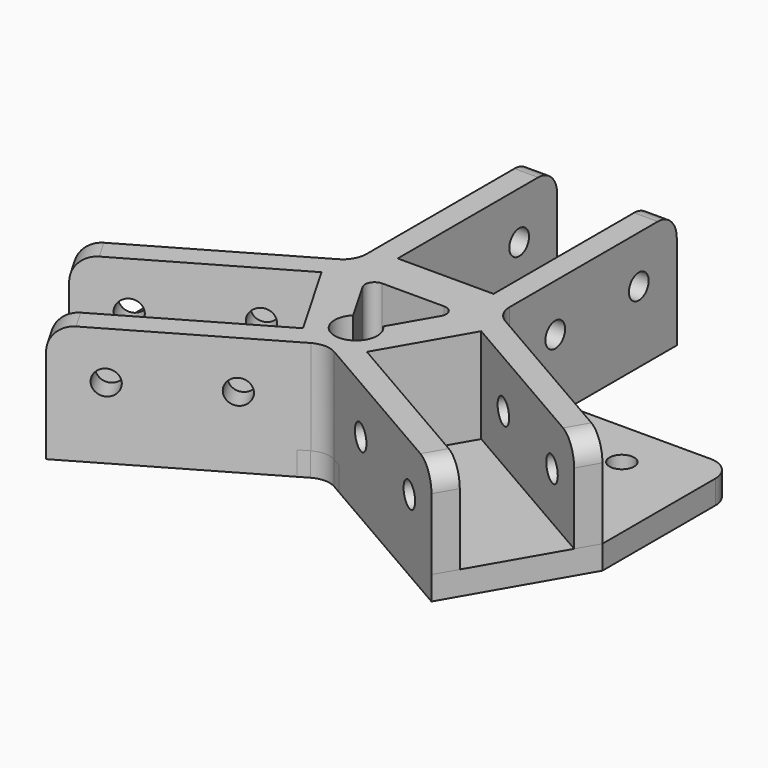
from build123d import *

# Parameters (mm, degrees)
F1_DEPTH    = 20
F2_R        = 2.6
F3_DEPTH    = 50.6016350946
F4_COUNT    = 3
F4_ANGLE    = 240
F6_DEPTH    = 5
F7_T1_DEPTH = 25
F10_DEPTH   = 5
F11_DEPTH   = 25.001
F12_R       = 2
F13_R       = 2.6
F14_DEPTH   = 25.001
F15_R       = 5
F16_R       = 4.5
F17_DEPTH   = 20


# Not quite as in the source:
# - a fillet or chamfer that OpenCascade refuses, or shapes differently, is made with other operations: its cross-section is extruded or revolved along the edge and cut away or added


with BuildPart() as f1:
    # F0 (on Top) → F1 (new body)
    with BuildSketch(Plane.XY):
        Polygon((43.0992290895, -36.5458269543), (6.7261621305, -15.5458269543), (16.8261621305, 1.9478862021), (53.1992290895, -19.0521137979), (55.6992290895, -14.7219867789), (14.8979589003, 8.8346375481), (0, 0), (-0.2020410997, -17.3193296462), (40.5992290895, -40.8759539732), align=None)
    extrude(amount=F1_DEPTH)

    # F2 (on face) → F3 (cut, through all)
    with BuildSketch(Plane(origin=(-7.55, -13.0769835971, 0), x_dir=(0.8660254038, -0.5, 0), z_dir=(-0.5, -0.8660254038, 0))):
        with Locations((45.5979407522, 10)):
            Circle(F2_R)
        with Locations((23.5979407522, 10)):
            Circle(F2_R)
    extrude(amount=-F3_DEPTH, mode=Mode.SUBTRACT)

    # F4: F1 ×3 about axis
    f4_axis = Axis((0, 0, 10), (0, 0, -1))


with BuildPart() as f1_1:
    add(f1.part)
    for i in range(1, F4_COUNT):
        add(f1.part.rotate(f4_axis, i * F4_ANGLE / (F4_COUNT - 1)))

    # F5 (on face) → F6 (join)
    with BuildSketch(Plane(origin=(0, 0, 0), x_dir=(1, 0, 0), z_dir=(0, 0, -1))):
        Polygon((0, 17.4359781295), (-40.5992290895, 40.8759539732), (-55.6992290895, 14.7219867789), (-15.1, -8.7179890648), (-15.1, -55.5979407522), (15.1, -55.5979407522), (15.1, -8.7179890648), (55.6992290895, 14.7219867789), (40.5992290895, 40.8759539732), align=None)
    extrude(amount=F6_DEPTH)

    # F7: fillet of radius 5 on 3 edges, made by hand

    # F7_s2 → F7_t1 (join)
    with BuildSketch(Plane.XY.offset(-5)):
        with BuildLine():
            ThreePointArc((2.5012, -18.8795847426), (0, -18.2093902225), (-2.5012, -18.8795847426))
            Line((-2.5012, -18.8795847426), (-2.75132, -18.4463641946))
            ThreePointArc((-2.75132, -18.4463641946), (-1.50062, -17.7247340932), (-0.25012, -17.0027575815))
            Line((-0.25012, -17.0027575815), (0.25012, -17.0027575815))
            ThreePointArc((0.25012, -17.0027575815), (1.50062, -17.7247340932), (2.75132, -18.4463641946))
            Line((2.75132, -18.4463641946), (2.5012, -18.8795847426))
        make_face()
        with BuildLine():
            ThreePointArc((15.0996, 11.6058951112), (15.7697945201, 9.1046951112), (17.6008, 7.2736896314))
            Line((17.6008, 7.2736896314), (17.35068, 6.8404690834))
            ThreePointArc((17.35068, 6.8404690834), (16.10038, 7.5627920052), (14.84988, 8.2847685168))
            Line((14.84988, 8.2847685168), (14.59976, 8.7179890648))
            ThreePointArc((14.59976, 8.7179890648), (14.59976, 10.161942088), (14.59936, 11.6058951112))
            Line((14.59936, 11.6058951112), (15.0996, 11.6058951112))
        make_face()
        with BuildLine():
            ThreePointArc((-17.6008, 7.2736896314), (-15.7697945201, 9.1046951112), (-15.0996, 11.6058951112))
            Line((-15.0996, 11.6058951112), (-14.59936, 11.6058951112))
            ThreePointArc((-14.59936, 11.6058951112), (-14.59976, 10.161942088), (-14.59976, 8.7179890648))
            Line((-14.59976, 8.7179890648), (-14.84988, 8.2847685168))
            ThreePointArc((-14.84988, 8.2847685168), (-16.10038, 7.5627920052), (-17.35068, 6.8404690834))
            Line((-17.35068, 6.8404690834), (-17.6008, 7.2736896314))
        make_face()
    extrude(amount=F7_T1_DEPTH)

    # F9 (on face) → F10 (join)
    with BuildSketch(Plane(origin=(0, 0, -5), x_dir=(1, 0, 0), z_dir=(0, 0, -1))):
        with BuildLine():
            Line((-55.6992290895, 14.7219867789), (-55.6992290895, -20))
            Line((-55.6992290895, -20), (55.6992290895, -20))
            Line((55.6992290895, -20), (55.6992290895, 14.7219867789))
            Line((55.6992290895, 14.7219867789), (52.6519667355, 20))
            Line((52.6519667355, 20), (4.4410161514, 20))
            Line((4.4410161514, 20), (2.5, 18.8793538025))
            ThreePointArc((2.5, 18.8793538025), (0, 18.2094808214), (-2.5, 18.8793538025))
            Line((-2.5, 18.8793538025), (-4.4410161514, 20))
            Line((-4.4410161514, 20), (-52.6519667355, 20))
            Line((-52.6519667355, 20), (-55.6992290895, 14.7219867789))
        make_face()
    extrude(amount=-F10_DEPTH)

    # F8 (on face) → F11 (cut, through all)
    with BuildSketch(Plane.XY.offset(20)):
        Polygon((10, 5.0614941438), (-10, 5.0614941438), (0, -12.2590139319), align=None)
    extrude(amount=-F11_DEPTH, mode=Mode.SUBTRACT)

    # F12
    f12_edges = [f1_1.edges().sort_by_distance(p)[0] for p in [
        (10, 5.061494, 7.5),
        (-10, 5.061494, 7.5),
        (0, -12.259014, 7.5),
    ]]
    fillet(f12_edges, radius=F12_R)

    # F13 (on face) → F14 (cut, through all)
    with BuildSketch(Plane(origin=(0, 0, -5), x_dir=(1, 0, 0), z_dir=(0, 0, -1))):
        with Locations((-40, -10)):
            Circle(F13_R)
        with Locations((40, -10)):
            Circle(F13_R)
        with Locations((0, 10)):
            Circle(F13_R)
    extrude(amount=-F14_DEPTH, mode=Mode.SUBTRACT)

    # F15
    f15_edges = [f1_1.edges().sort_by_distance(p)[0] for p in [
        (-15.1, 20, -2.5),
        (15.1, 20, -2.5),
        (55.699229, 20, -2.5),
        (-55.699229, 20, -2.5),
        (-12.6, 55.597941, 20),
        (12.6, 55.597941, 20),
        (-54.449229, -16.88705, 20),
        (-41.849229, -38.71089, 20),
        (54.449229, -16.88705, 20),
        (41.849229, -38.71089, 20),
    ]]
    fillet(f15_edges, radius=F15_R)

    # F16 (on face) → F17 (cut)
    with BuildSketch(Plane.XY.offset(20)):
        with Locations((0, -10)):
            Circle(F16_R)
    extrude(amount=-F17_DEPTH, mode=Mode.SUBTRACT)


solid = f1_1.part
